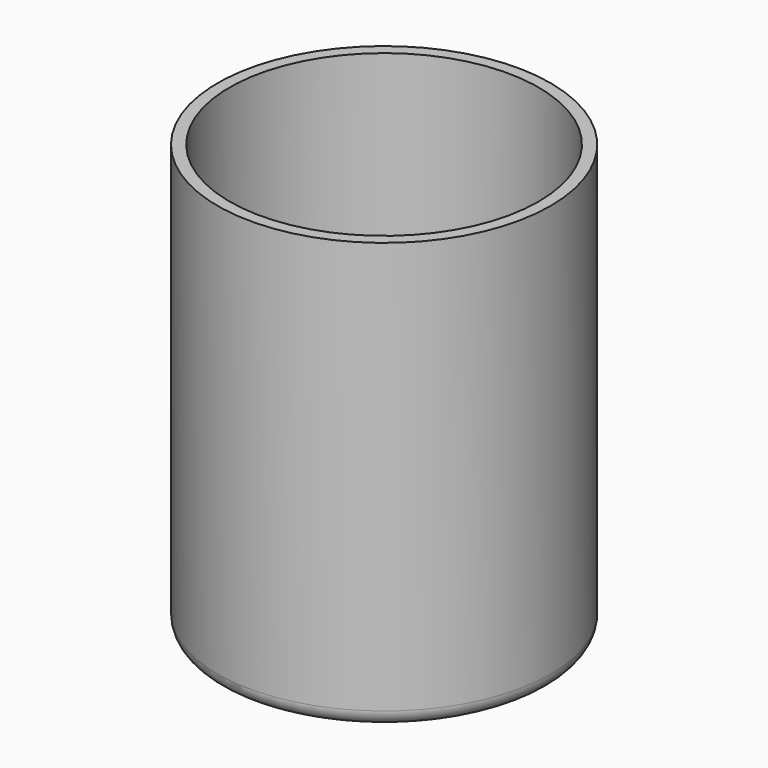
from build123d import *

# Parameters (mm, degrees)
F0_R            = 266.7
F0_R_2          = 247.65
F1_DEPTH        = 635
F2_R            = 266.7
F3_DEPTH        = 50.8
F4_R            = 25.4
F5_R            = 38.1
F7_DEPTH        = 50.8
F7_COPIES_COUNT = 8
F8_R            = 31.75
F9_DEPTH        = 50.8


# Not quite as in the source:
# - a pattern or mirror of a feature is missing from the dataset's text; its kind, count and spacing are read off the source's solid
# - a feature names something its author has since deleted; it is built from what else it names


with BuildPart() as f1:
    # F0 (on Top) → F1 (new body)
    with BuildSketch(Plane.XY):
        Circle(F0_R)
        Circle(F0_R_2, mode=Mode.SUBTRACT)
    extrude(amount=F1_DEPTH)

    # F2 (on face) → F3 (join)
    with BuildSketch(Plane(origin=(0, 0, 0), x_dir=(1, 0, 0), z_dir=(0, 0, -1))):
        Circle(F2_R)
    extrude(amount=F3_DEPTH)

    # F4
    f4_edges = [f1.edges().sort_by_distance(p)[0] for p in [
        (-266.7, 0, -50.8),
    ]]
    fillet(f4_edges, radius=F4_R)

    # F5 (on face) → F7 (cut, through all)
    with BuildSketch(Plane(origin=(0, 0, -50.8), x_dir=(1, 0, 0), z_dir=(0, 0, -1))):
        with Locations((-177.8, 0)):
            Circle(F5_R)
    f7 = extrude(amount=-F7_DEPTH, mode=Mode.SUBTRACT)

    # F7_copies: F7 ×8 about axis
    f7_copies_axis = Axis((0, 0, 0), (0, 0, 1))
    for i in range(1, F7_COPIES_COUNT):
        add(f7.rotate(f7_copies_axis, i * 360 / F7_COPIES_COUNT), mode=Mode.SUBTRACT)

    # F8 (on face) → F9 (cut, through all)
    with BuildSketch(Plane(origin=(0, 0, -50.8), x_dir=(1, 0, 0), z_dir=(0, 0, -1))):
        with Locations((0, 66.04)):
            Circle(F8_R)
        with Locations((66.04, 0)):
            Circle(F8_R)
        with Locations((-66.04, 0)):
            Circle(F8_R)
        with Locations((0, -66.04)):
            Circle(F8_R)
    extrude(amount=-F9_DEPTH, mode=Mode.SUBTRACT)


solid = f1.part
